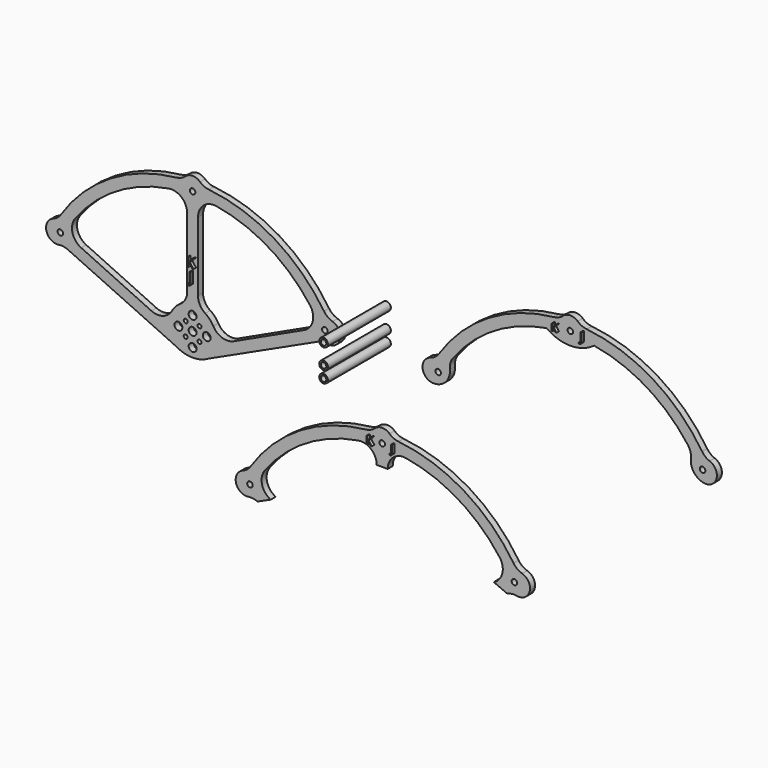
from build123d import *

# Parameters (mm, degrees)
F0_R           = 2.5
F0_R_2         = 1.25
F0_R_3         = 1.75
F1_DEPTH       = 4
F2_TEXT_SIZE   = 7.7073151867
F2_TEXT_SIZE_2 = 8.8418626951
F3_DEPTH       = 6
F4_TEXT_SIZE   = 5.9586432245
F4_TEXT_SIZE_2 = 7.4963654495
F5_DEPTH       = 6
F6_R           = 2.75
F6_R_2         = 1.75
F7_DEPTH       = 50
F9_TEXT_SIZE   = 6.7679935859
F9_TEXT_SIZE_2 = 6.8330723378
F10_DEPTH      = 2


# Not quite as in the source:
# - ends of sketch curves that miss each other by under 0.0002 mm in the source are joined
# - Text() gives the source's letters only with a copy of the font that has no kerning and outlines rounded to 1/6400 em; it was checked with that copy


with BuildPart() as f1:
    # F0 (on Front) → F1 (new body)
    with BuildSketch(Plane.XZ):
        with BuildLine():
            ThreePointArc((-109.6373380269, 43.9548487414), (-112.6732536981, 44.766978356), (-115.3071962011, 46.4812377774))
            ThreePointArc((-115.3071962011, 46.4812377774), (-120, 48.287242), (-124.6928038166, 46.481237797))
            ThreePointArc((-124.6928038166, 46.481237797), (-127.3267463019, 44.766978356), (-130.3626619731, 43.9548487414))
            ThreePointArc((-130.3626619731, 43.9548487414), (-172.0205091137, 29.9311746777), (-203.668843183, -0.5716548794))
            ThreePointArc((-203.668843183, -0.5716548794), (-205.7890431816, -2.891372583), (-208.524497209, -4.4385084396))
            ThreePointArc((-208.524497209, -4.4385084396), (-212.8537295752, -12.7573359601), (-205.0229859426, -17.9172383762))
            ThreePointArc((-205.0229859426, -17.9172383762), (-202.0950101693, -17.9042009353), (-199.2887689394, -18.73979787))
            Line((-199.2887689394, -18.73979787), (-130, -50.712758))
            ThreePointArc((-130, -50.712758), (-120, -53.409448), (-109.9999999125, -50.7127581505))
            Line((-109.9999999125, -50.7127581505), (-40.5819451393, -18.6801396786))
            ThreePointArc((-40.5819451393, -18.6801396786), (-40.5337321435, -18.6571856673), (-40.485397265, -18.6344894316))
            ThreePointArc((-40.485397265, -18.6344894316), (-37.4974000092, -17.7745183048), (-34.3896989177, -17.8738755677))
            ThreePointArc((-34.3896989177, -17.8738755677), (-26.2800031592, -12.654371205), (-31.0798389877, -4.2894459589))
            ThreePointArc((-31.0798389877, -4.2894459589), (-34.1691835034, -2.7453971145), (-36.5490183316, -0.2424942204))
            ThreePointArc((-36.5490183316, -0.2424942204), (-68.1482765915, 30.0334684622), (-109.6373380269, 43.9548487414))
        make_face()
        with Locations((-120, -47.712758)):
            Circle(F0_R, mode=Mode.SUBTRACT)
        with Locations((-124.384062, -43.09682)):
            Circle(F0_R_2, mode=Mode.SUBTRACT)
        with Locations((-115.615938, -43.09682)):
            Circle(F0_R_2, mode=Mode.SUBTRACT)
        with Locations((-129, -38.712758)):
            Circle(F0_R, mode=Mode.SUBTRACT)
        with Locations((-120, -38.712758)):
            Circle(F0_R, mode=Mode.SUBTRACT)
        with Locations((-111, -38.712758)):
            Circle(F0_R, mode=Mode.SUBTRACT)
        with Locations((-124.384062, -34.328696)):
            Circle(F0_R_2, mode=Mode.SUBTRACT)
        with Locations((-115.615938, -34.328696)):
            Circle(F0_R_2, mode=Mode.SUBTRACT)
        with Locations((-120, -29.712758)):
            Circle(F0_R, mode=Mode.SUBTRACT)
        with Locations((-204, -10.712758)):
            Circle(F0_R_3, mode=Mode.SUBTRACT)
        with BuildLine():
            ThreePointArc((-133.1498130132, -31.4959429927), (-138.8025603315, -36.187589558), (-146.1356700483, -35.7510101038))
            Line((-146.1356700483, -35.7510101038), (-190.847957, -14.942553))
            ThreePointArc((-190.847957, -14.942553), (-196.3263434158, -8.316478297), (-194.6364231411, 0.1133351056))
            ThreePointArc((-194.6364231411, 0.1133351056), (-168.3733961758, 23.9563256735), (-135.1040320231, 36.2601541404))
            ThreePointArc((-135.1040320231, 36.2601541404), (-127.0163589939, 34.0196460136), (-123.4835240454, 26.407195))
            Line((-123.4835240454, 26.407195), (-123.418107, -17.603945))
            ThreePointArc((-123.418107, -17.603945), (-124.6488960109, -22.4251726516), (-128.0508580001, -26.0563889998))
            ThreePointArc((-128.0508580001, -26.0563889998), (-130.9436877656, -28.4543127918), (-133.1498130132, -31.4959429927))
        make_face(mode=Mode.SUBTRACT)
        with BuildLine():
            Line((-49.152043, -14.942553), (-93.86433, -35.75101))
            ThreePointArc((-93.86433, -35.75101), (-101.1974396685, -36.187589558), (-106.8501869868, -31.4959429927))
            ThreePointArc((-106.8501869868, -31.4959429927), (-109.0563099527, -28.4543152259), (-111.9491362053, -26.0563923227))
            ThreePointArc((-111.9491362053, -26.0563923227), (-115.3510979946, -22.425169519), (-116.5818819308, -17.6039360001))
            Line((-116.5818819308, -17.6039360001), (-116.516396, 26.407198))
            ThreePointArc((-116.516396, 26.407198), (-112.9835510174, 34.0196414829), (-104.8958778849, 36.260139701))
            ThreePointArc((-104.8958778849, 36.260139701), (-71.626564829, 23.9563019963), (-45.363576772, 0.1133351705))
            ThreePointArc((-45.363576772, 0.1133351705), (-43.6736565842, -8.316478297), (-49.152043, -14.942553))
        make_face(mode=Mode.SUBTRACT)
        with Locations((-36, -10.712758)):
            Circle(F0_R_3, mode=Mode.SUBTRACT)
        with Locations((-120, 39.581523)):
            Circle(F0_R_3, mode=Mode.SUBTRACT)
    extrude(amount=F1_DEPTH)

    # F2 (on Front) → F3 (join)
    with BuildSketch(Plane.XZ):
        with Locations((-122.5709468126, -2.3656911217)):
            Text('K', F2_TEXT_SIZE, font='Open Sans', text_align=(TextAlign.LEFT, TextAlign.BOTTOM))
        with Locations((-121.1595907807, -11.0068460926)):
            Text('J', F2_TEXT_SIZE_2, font='Open Sans', text_align=(TextAlign.LEFT, TextAlign.BOTTOM))
    extrude(amount=F3_DEPTH)


with BuildPart() as f1b:
    # F0 (on Front) → F1, piece 2 (new body)
    with BuildSketch(Plane.XZ):
        with BuildLine():
            ThreePointArc((45.363576772, 0.1133351705), (71.626564829, 23.9563019963), (104.8958779418, 36.2601393546))
            ThreePointArc((104.8958779418, 36.2601393546), (119.9999574997, 31.287242), (135.1040320915, 36.2601538762))
            ThreePointArc((135.1040320915, 36.2601538762), (168.3733961758, 23.9563256735), (194.636423228, 0.1133351705))
            ThreePointArc((194.636423228, 0.1133351705), (196.2738224848, -3.2361067979), (196.5705573976, -6.9525279348))
            ThreePointArc((196.5705573976, -6.9525279348), (198.589673296, -14.1303572428), (205.0137120202, -17.915827867))
            ThreePointArc((205.0137120202, -17.915827867), (205.0183491243, -17.9165321824), (205.022985938, -17.9172384067))
            ThreePointArc((205.022985938, -17.9172384067), (212.8537295752, -12.7573359601), (208.5244970585, -4.4385088432))
            ThreePointArc((208.5244970585, -4.4385088432), (205.7890431816, -2.891372583), (203.6688433214, -0.5716547882))
            ThreePointArc((203.6688433214, -0.5716547882), (172.0205091137, 29.9311746777), (130.3626619608, 43.9548486234))
            ThreePointArc((130.3626619608, 43.9548486234), (127.3267463019, 44.766978356), (124.6928037989, 46.4812377774))
            ThreePointArc((124.6928037989, 46.4812377774), (120, 48.287242), (115.3071961834, 46.481237797))
            ThreePointArc((115.3071961834, 46.481237797), (112.6732536981, 44.766978356), (109.6373380269, 43.9548487414))
            ThreePointArc((109.6373380269, 43.9548487414), (68.1482765915, 30.0334684622), (36.5490180501, -0.2424940333))
            ThreePointArc((36.5490180501, -0.2424940333), (34.1691835034, -2.7453971145), (31.0798390683, -4.289446229))
            ThreePointArc((31.0798390683, -4.289446229), (26.2800031592, -12.654371205), (34.38969902, -17.8738761049))
            ThreePointArc((34.38969902, -17.8738761049), (34.5024750937, -17.8514527387), (34.6148676335, -17.8271799729))
            ThreePointArc((34.6148676335, -17.8271799729), (41.2634218878, -14.1625861594), (43.4223048074, -6.8844170195))
            ThreePointArc((43.4223048074, -6.8844170195), (43.7352745151, -3.2030952967), (45.363576772, 0.1133351705))
        make_face()
        with Locations((36, -10.712758)):
            Circle(F0_R_3, mode=Mode.SUBTRACT)
        with Locations((204, -10.712758)):
            Circle(F0_R_3, mode=Mode.SUBTRACT)
        with Locations((120, 39.581523)):
            Circle(F0_R_3, mode=Mode.SUBTRACT)
    extrude(amount=F1_DEPTH)

    # F4 (on Front) → F5 (join)
    with BuildSketch(Plane.XZ):
        with Locations((109.1276481748, 37.0230264962)):
            Text('K', F4_TEXT_SIZE, font='Open Sans', text_align=(TextAlign.LEFT, TextAlign.BOTTOM))
        with Locations((127.2573247552, 36.8846282363)):
            Text('J', F4_TEXT_SIZE_2, font='Open Sans', text_align=(TextAlign.LEFT, TextAlign.BOTTOM))
    extrude(amount=F5_DEPTH)


with BuildPart() as f1c:
    # F0 (on Front) → F1, piece 3 (new body)
    with BuildSketch(Plane.XZ):
        with BuildLine():
            ThreePointArc((15.5512461315, -65.498796331), (48.8205592443, -77.8026336892), (75.0835473013, -101.6456005151))
            ThreePointArc((75.0835473013, -101.6456005151), (76.7734674891, -110.0754139826), (71.2950811216, -116.7014887894))
            Line((71.2950811216, -116.7014887894), (79.9617268083, -120.3934251172))
            ThreePointArc((79.9617268083, -120.3934251172), (82.9497240641, -119.5334539904), (86.0574251556, -119.6328112533))
            ThreePointArc((86.0574251556, -119.6328112533), (94.1671209141, -114.4133068906), (89.3672850855, -106.0483816445))
            ThreePointArc((89.3672850855, -106.0483816445), (86.2779405699, -104.5043328001), (83.8981057417, -102.001429906))
            ThreePointArc((83.8981057417, -102.001429906), (52.2988474818, -71.7254672233), (10.8097860341, -57.8040870622))
            ThreePointArc((10.8097860341, -57.8040870622), (7.7738703752, -56.9919573296), (5.1399278722, -55.2776979082))
            ThreePointArc((5.1399278722, -55.2776979082), (0.4471240733, -53.4716936856), (-4.2456797433, -55.2776978886))
            ThreePointArc((-4.2456797433, -55.2776978886), (-6.8796222286, -56.9919573296), (-9.9155378998, -57.8040869442))
            ThreePointArc((-9.9155378998, -57.8040869442), (-51.5733850404, -71.8277610079), (-83.2217191097, -102.3305905649))
            ThreePointArc((-83.2217191097, -102.3305905649), (-85.3419191083, -104.6503082686), (-88.0773731357, -106.1974441251))
            ThreePointArc((-88.0773731357, -106.1974441251), (-92.4066055019, -114.5162716456), (-84.5758618693, -119.6761740618))
            ThreePointArc((-84.5758618693, -119.6761740618), (-81.647886096, -119.6631366208), (-78.8416448661, -120.4987335556))
            Line((-78.8416448661, -120.4987335556), (-70.4008329267, -116.7014886856))
            ThreePointArc((-70.4008329267, -116.7014886856), (-75.8792193425, -110.0754139826), (-74.1892990678, -101.64560058))
            ThreePointArc((-74.1892990678, -101.64560058), (-47.9262721025, -77.8026100121), (-14.6569079498, -65.4987815451))
            ThreePointArc((-14.6569079498, -65.4987815451), (-6.5692349206, -67.739289672), (-3.0363999722, -75.3517406856))
            Line((-3.0363999722, -75.3517406856), (3.9307281425, -75.3517376857))
            ThreePointArc((3.9307281425, -75.3517376857), (7.4635730559, -67.7392942027), (15.5512461315, -65.498796331))
        make_face()
        with Locations((-83.5528759267, -112.4716936856)):
            Circle(F0_R_3, mode=Mode.SUBTRACT)
        with Locations((84.4471240733, -112.4716936856)):
            Circle(F0_R_3, mode=Mode.SUBTRACT)
        with Locations((0.4471240733, -62.1774126856)):
            Circle(F0_R_3, mode=Mode.SUBTRACT)
    extrude(amount=F1_DEPTH)

    # F9 (on face) → F10 (join)
    with BuildSketch(Plane.XZ.offset(4)):
        with Locations((-8.6780944839, -64.6390318871)):
            Text('K', F9_TEXT_SIZE, font='Open Sans', text_align=(TextAlign.LEFT, TextAlign.BOTTOM))
        with Locations((7.1121579967, -64.5453259349)):
            Text('J', F9_TEXT_SIZE_2, font='Open Sans', text_align=(TextAlign.LEFT, TextAlign.BOTTOM))
    extrude(amount=F10_DEPTH)


with BuildPart() as f7:
    # F6 (on Front) → F7 (new body)
    with BuildSketch(Plane.XZ):
        Circle(F6_R)
        Circle(F6_R_2, mode=Mode.SUBTRACT)
    extrude(amount=F7_DEPTH)


with BuildPart() as f7b:
    # F6 (on Front) → F7, piece 2 (new body)
    with BuildSketch(Plane.XZ):
        with Locations((0, 12.8003004938)):
            Circle(F6_R)
        with Locations((0, 12.8003004938)):
            Circle(F6_R_2, mode=Mode.SUBTRACT)
    extrude(amount=F7_DEPTH)


with BuildPart() as f7c:
    # F6 (on Front) → F7, piece 3 (new body)
    with BuildSketch(Plane.XZ):
        with Locations((0, -7.390675135)):
            Circle(F6_R)
        with Locations((0, -7.390675135)):
            Circle(F6_R_2, mode=Mode.SUBTRACT)
    extrude(amount=F7_DEPTH)


with BuildPart() as f7d:
    # F6 (on Front) → F7, piece 4 (new body)
    with BuildSketch(Plane.XZ):
        with Locations((0, -20.4417593777)):
            Circle(F6_R)
        with Locations((0, -20.4417593777)):
            Circle(F6_R_2, mode=Mode.SUBTRACT)
    extrude(amount=F7_DEPTH)


solid = Compound([f1.part, f1b.part, f1c.part, f7.part, f7b.part, f7c.part])
